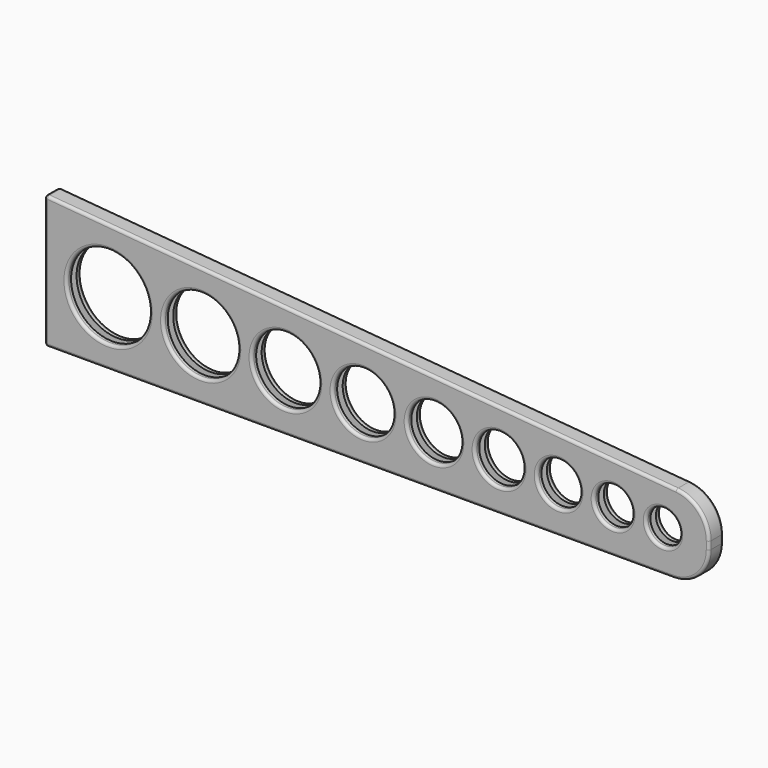
from build123d import *

# Parameters (mm, degrees)
F0_W     = 3
F0_H     = 42
F0_R     = 15.0407454206
F0_R_2   = 13.5592924796
F0_R_3   = 12.2029598094
F0_R_4   = 10.9611800259
F0_R_5   = 8.7833966951
F0_R_6   = 9.8242782432
F0_R_7   = 7.8304257228
F0_R_8   = 6.9579405917
F0_R_9   = 6.1591436438
F1_DEPTH = 2
F2_DEPTH = 4.5
F3_START = 4.5
F3_DEPTH = 2
F4_SIZE  = 1
F5_R     = 0.99999


# Not quite as in the source:
# - a fillet or chamfer is up to 0.001 mm smaller than in the source, because OpenCascade refuses the exact size


with BuildPart() as f1:
    # F0 (on Front) → F1 (new body)
    with BuildSketch(Plane.XZ):
        with Locations((-121.7048612587, 21)):
            Rectangle(F0_W, F0_H)
        with BuildLine():
            Line((104.7951387413, 0), (-120.2048612587, 0))
            Line((-120.2048612587, 0), (-123.2048612587, 0))
            Line((-123.2048612587, 0), (-123.2048612587, -3))
            Line((-123.2048612587, -3), (104.7951387413, -3))
            ThreePointArc((104.7951387413, -3), (113.9875268967, 0.8076118446), (117.7951387413, 10))
            Line((117.7951387413, 10), (117.7951387413, 12.8149136893))
            ThreePointArc((117.7951387413, 12.8149136893), (114.3693533654, 21.6089124573), (105.8975365365, 25.768087783))
            Line((105.8975365365, 25.768087783), (-123.2048612587, 45.2661641911))
            Line((-123.2048612587, 45.2661641911), (-123.2048612587, 42))
            Line((-123.2048612587, 42), (-120.2048612587, 42))
            Line((-120.2048612587, 42), (105.6431370453, 22.7788937614))
            ThreePointArc((105.6431370453, 22.7788937614), (112.1599192214, 19.5795281262), (114.7951387413, 12.8149136893))
            Line((114.7951387413, 12.8149136893), (114.7951387413, 10))
            ThreePointArc((114.7951387413, 10), (111.8662065532, 2.9289321881), (104.7951387413, 0))
        make_face()
        with BuildLine():
            Line((-120.2048612587, 42), (-120.2048612587, 0))
            Line((-120.2048612587, 0), (104.7951387413, 0))
            ThreePointArc((104.7951387413, 0), (111.8662065532, 2.9289321881), (114.7951387413, 10))
            Line((114.7951387413, 10), (114.7951387413, 12.8149136893))
            ThreePointArc((114.7951387413, 12.8149136893), (112.1599192214, 19.5795281262), (105.6431370453, 22.7788937614))
            Line((105.6431370453, 22.7788937614), (-120.2048612587, 42))
        make_face()
        with Locations((-100.180791127, 20.1826308218)):
            Circle(F0_R, mode=Mode.SUBTRACT)
        with Locations((-66.6087107866, 18.8122409091)):
            Circle(F0_R_2, mode=Mode.SUBTRACT)
        with Locations((-35.8720548232, 17.557591127)):
            Circle(F0_R_3, mode=Mode.SUBTRACT)
        with Locations((-7.7313495038, 16.4089063177)):
            Circle(F0_R_4, mode=Mode.SUBTRACT)
        with Locations((41.6206851942, 14.3943892001)):
            Circle(F0_R_5, mode=Mode.SUBTRACT)
        with Locations((18.0326534773, 15.3572369115)):
            Circle(F0_R_6, mode=Mode.SUBTRACT)
        with Locations((63.2165234141, 13.5128614975)):
            Circle(F0_R_7, mode=Mode.SUBTRACT)
        with Locations((82.9884244366, 12.705785694)):
            Circle(F0_R_8, mode=Mode.SUBTRACT)
        with Locations((101.0904340027, 11.9668737452)):
            Circle(F0_R_9, mode=Mode.SUBTRACT)
    extrude(amount=F1_DEPTH)

    # F0 (on Front) → F2 (join)
    with BuildSketch(Plane.XZ):
        with BuildLine():
            Line((104.7951387413, 0), (-120.2048612587, 0))
            Line((-120.2048612587, 0), (-123.2048612587, 0))
            Line((-123.2048612587, 0), (-123.2048612587, -3))
            Line((-123.2048612587, -3), (104.7951387413, -3))
            ThreePointArc((104.7951387413, -3), (113.9875268967, 0.8076118446), (117.7951387413, 10))
            Line((117.7951387413, 10), (117.7951387413, 12.8149136893))
            ThreePointArc((117.7951387413, 12.8149136893), (114.3693533654, 21.6089124573), (105.8975365365, 25.768087783))
            Line((105.8975365365, 25.768087783), (-123.2048612587, 45.2661641911))
            Line((-123.2048612587, 45.2661641911), (-123.2048612587, 42))
            Line((-123.2048612587, 42), (-120.2048612587, 42))
            Line((-120.2048612587, 42), (105.6431370453, 22.7788937614))
            ThreePointArc((105.6431370453, 22.7788937614), (112.1599192214, 19.5795281262), (114.7951387413, 12.8149136893))
            Line((114.7951387413, 12.8149136893), (114.7951387413, 10))
            ThreePointArc((114.7951387413, 10), (111.8662065532, 2.9289321881), (104.7951387413, 0))
        make_face()
    extrude(amount=F2_DEPTH)

    # F0 (on Front) → F3 (join)
    with BuildSketch(Plane.XZ.offset(F3_START)):
        with BuildLine():
            Line((104.7951387413, 0), (-120.2048612587, 0))
            Line((-120.2048612587, 0), (-123.2048612587, 0))
            Line((-123.2048612587, 0), (-123.2048612587, -3))
            Line((-123.2048612587, -3), (104.7951387413, -3))
            ThreePointArc((104.7951387413, -3), (113.9875268967, 0.8076118446), (117.7951387413, 10))
            Line((117.7951387413, 10), (117.7951387413, 12.8149136893))
            ThreePointArc((117.7951387413, 12.8149136893), (114.3693533654, 21.6089124573), (105.8975365365, 25.768087783))
            Line((105.8975365365, 25.768087783), (-123.2048612587, 45.2661641911))
            Line((-123.2048612587, 45.2661641911), (-123.2048612587, 42))
            Line((-123.2048612587, 42), (-120.2048612587, 42))
            Line((-120.2048612587, 42), (105.6431370453, 22.7788937614))
            ThreePointArc((105.6431370453, 22.7788937614), (112.1599192214, 19.5795281262), (114.7951387413, 12.8149136893))
            Line((114.7951387413, 12.8149136893), (114.7951387413, 10))
            ThreePointArc((114.7951387413, 10), (111.8662065532, 2.9289321881), (104.7951387413, 0))
        make_face()
        with Locations((-121.7048612587, 21)):
            Rectangle(F0_W, F0_H)
        with BuildLine():
            Line((-120.2048612587, 42), (-120.2048612587, 0))
            Line((-120.2048612587, 0), (104.7951387413, 0))
            ThreePointArc((104.7951387413, 0), (111.8662065532, 2.9289321881), (114.7951387413, 10))
            Line((114.7951387413, 10), (114.7951387413, 12.8149136893))
            ThreePointArc((114.7951387413, 12.8149136893), (112.1599192214, 19.5795281262), (105.6431370453, 22.7788937614))
            Line((105.6431370453, 22.7788937614), (-120.2048612587, 42))
        make_face()
        with Locations((-100.180791127, 20.1826308218)):
            Circle(F0_R, mode=Mode.SUBTRACT)
        with Locations((-66.6087107866, 18.8122409091)):
            Circle(F0_R_2, mode=Mode.SUBTRACT)
        with Locations((-35.8720548232, 17.557591127)):
            Circle(F0_R_3, mode=Mode.SUBTRACT)
        with Locations((-7.7313495038, 16.4089063177)):
            Circle(F0_R_4, mode=Mode.SUBTRACT)
        with Locations((41.6206851942, 14.3943892001)):
            Circle(F0_R_5, mode=Mode.SUBTRACT)
        with Locations((18.0326534773, 15.3572369115)):
            Circle(F0_R_6, mode=Mode.SUBTRACT)
        with Locations((63.2165234141, 13.5128614975)):
            Circle(F0_R_7, mode=Mode.SUBTRACT)
        with Locations((82.9884244366, 12.705785694)):
            Circle(F0_R_8, mode=Mode.SUBTRACT)
        with Locations((101.0904340027, 11.9668737452)):
            Circle(F0_R_9, mode=Mode.SUBTRACT)
    extrude(amount=F3_DEPTH)

    # F4
    f4_edges = [f1.edges().sort_by_distance(p)[0] for p in [
        (-123.204861, -4.5, 21),
        (-123.204861, -3.25, 0),
        (-123.204861, -2, 21),
        (-123.204861, -3.25, 42),
    ]]
    chamfer(f4_edges, length=F4_SIZE)

    # F5 (radius 1 in the source; OpenCascade refuses exactly that, so slightly less here)
    f5_edges = [f1.edges().sort_by_distance(p)[0] for p in [
        (-9.204861, 0, -3),
        (113.987527, 0, 0.807612),
        (117.795139, 0, 11.407457),
        (114.369353, 0, 21.608912),
        (-8.653662, 0, 35.517126),
        (-123.204861, 0, 21.133082),
        (94.93129, 0, 11.966874),
        (8.208375, 0, 15.357237),
        (32.837288, 0, 14.394389),
        (55.386098, 0, 13.512861),
        (76.030484, 0, 12.705786),
        (-115.221537, 0, 20.182631),
        (-80.168003, 0, 18.812241),
        (-18.69253, 0, 16.408906),
        (-48.075015, 0, 17.557591),
        (-9.204861, -6.5, -3),
        (113.987527, -6.5, 0.807612),
        (117.795139, -6.5, 11.407457),
        (114.369353, -6.5, 21.608912),
        (-8.653662, -6.5, 35.517126),
        (-123.204861, -6.5, 21.133082),
        (94.93129, -6.5, 11.966874),
        (-18.69253, -6.5, 16.408906),
        (32.837288, -6.5, 14.394389),
        (8.208375, -6.5, 15.357237),
        (55.386098, -6.5, 13.512861),
        (76.030484, -6.5, 12.705786),
        (-115.221537, -6.5, 20.182631),
        (-80.168003, -6.5, 18.812241),
        (-48.075015, -6.5, 17.557591),
        (-123.204861, -3.25, -3),
        (-123.204861, -3.25, 45.266164),
    ]]
    fillet(f5_edges, radius=F5_R)


solid = f1.part
